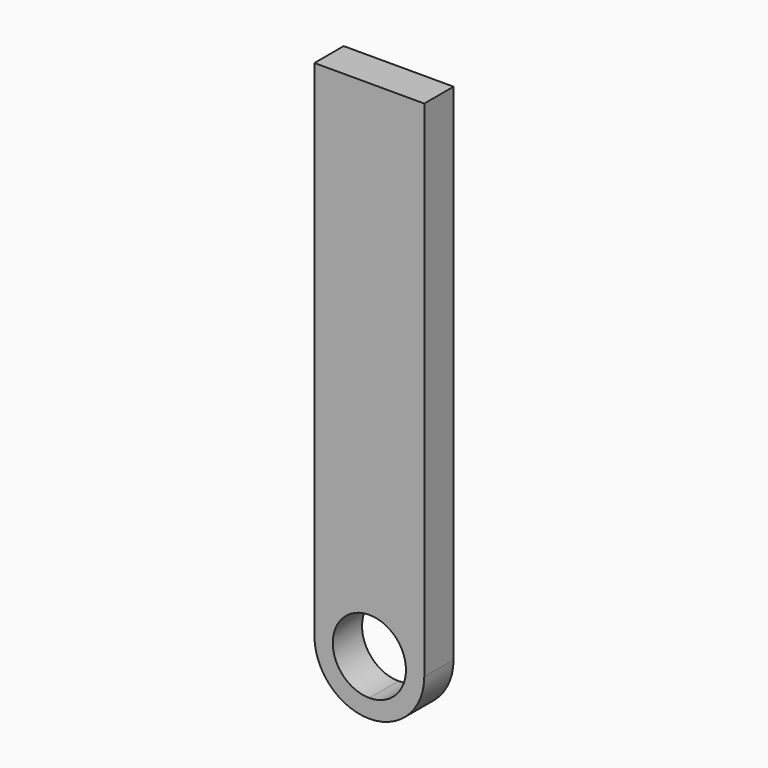
from build123d import *

# Parameters (mm, degrees)
F1_DEPTH = 3.175
F2_R     = 4.76249


# Not quite as in the source:
# - a fillet or chamfer is up to 0.001 mm smaller than in the source, because OpenCascade refuses the exact size


with BuildPart() as f1:
    # F0 (on Front) → F1 (new body)
    with BuildSketch(Plane.XZ):
        Polygon((0, 3.175), (0, 0), (0, -45.3541763127), (4.7625, -45.3541763127), (9.525, -45.3541763127), (9.525, 3.175), align=None)
        with BuildLine():
            ThreePointArc((7.9375, -40.5916763127), (7.0075640303, -42.836740343), (4.7625, -43.7666763127))
            ThreePointArc((4.7625, -43.7666763127), (2.5174359697, -38.3466122824), (7.9375, -40.5916763127))
        make_face(mode=Mode.SUBTRACT)
    extrude(amount=F1_DEPTH)

    # F2 (radius 4.7625 in the source; OpenCascade refuses exactly that, so slightly less here)
    f2_edges = [f1.edges().sort_by_distance(p)[0] for p in [
        (0, -1.5875, -45.354176),
        (9.525, -1.5875, -45.354176),
    ]]
    fillet(f2_edges, radius=F2_R)


solid = f1.part
